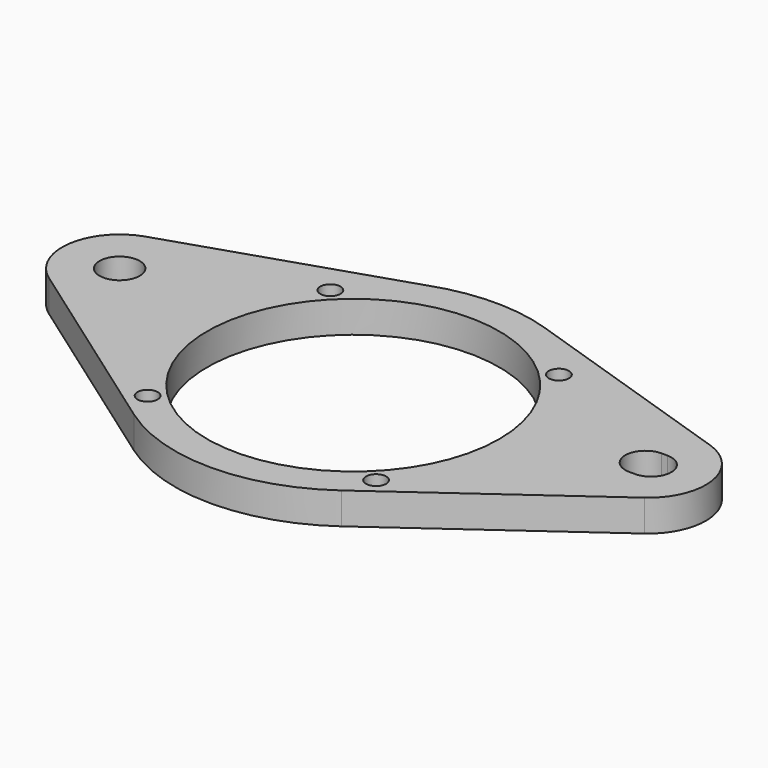
from build123d import *

# Parameters (mm, degrees)
F0_R      = 3.5
F0_R_2    = 25.4
F1_DEPTH  = 5.5
F2_DEPTH  = 33
F3_DEPTH  = 28
F4_R      = 2.5
F5_DEPTH  = 25.4
F6_R      = 5.08
F7_R      = 40.64
F8_DEPTH  = 33
F9_R      = 1.7526
F10_DEPTH = 5.501


with BuildPart() as f1:
    # F0 (on Top) → F1 (new body)
    with BuildSketch(Plane.XY):
        with BuildLine():
            Line((-3.3917498572, 9.4072330101), (-2.8084065037, 9.5975441082))
            ThreePointArc((-2.8084065037, 9.5975441082), (-3.1015382157, 9.5068638728), (-3.3917498572, 9.4072330101))
        make_face()
        with BuildLine():
            Line((35.7055754428, 22.1624223313), (-2.8084065037, 9.5975441082))
            Line((-2.8084065037, 9.5975441082), (-3.3917498572, 9.4072330101))
            ThreePointArc((-3.3917498572, 9.4072330101), (-9.9089012804, 1.3467276694), (-5.7794328291, -8.1607693371))
            Line((-5.7794328291, -8.1607693371), (28.3037582299, -32.2983849452))
            ThreePointArc((28.3037582299, -32.2983849452), (15.5024060308, -2.8251442248), (35.7055754428, 22.1624223313))
        make_face()
        Circle(F0_R, mode=Mode.SUBTRACT)
        with BuildLine():
            ThreePointArc((55.9525424009, 22.43259449), (45.80637798, 23.9972404711), (35.7055754428, 22.1624223313))
            ThreePointArc((35.7055754428, 22.1624223313), (15.5024060308, -2.8251442248), (28.3037582299, -32.2983849452))
            ThreePointArc((28.3037582299, -32.2983849452), (46.3284941146, -37.999810145), (64.3128808741, -32.1723590805))
            ThreePointArc((64.3128808741, -32.1723590805), (73.805134648, -21.1442690321), (77.22, -7))
            ThreePointArc((77.22, -7), (71.3467667481, 11.1561447666), (55.9525424009, 22.43259449))
        make_face()
        with Locations((46.22, -7)):
            Circle(F0_R_2, mode=Mode.SUBTRACT)
        with BuildLine():
            Line((95.0795298067, 9.4943853194), (55.9525424009, 22.43259449))
            ThreePointArc((55.9525424009, 22.43259449), (71.3467667481, 11.1561447666), (77.22, -7))
            ThreePointArc((77.22, -7), (73.805134648, -21.1442690321), (64.3128808741, -32.1723590805))
            Line((64.3128808741, -32.1723590805), (97.7764131852, -8.1201158324))
            ThreePointArc((97.7764131852, -8.1201158324), (101.8248141538, 1.5134229894), (95.0795298067, 9.4943853194))
        make_face()
        with BuildLine():
            ThreePointArc((91.44, -3.5), (87.94, 0), (91.44, 3.5))
            Line((91.44, 3.5), (92.44, 3.5))
            ThreePointArc((92.44, 3.5), (95.94, 0), (92.44, -3.5))
            Line((92.44, -3.5), (91.44, -3.5))
        make_face(mode=Mode.SUBTRACT)
    extrude(amount=F1_DEPTH)

    # F0 (on Top) → F2 (join)
    with BuildSketch(Plane.XY):
        with BuildLine():
            ThreePointArc((55.9525424009, 22.43259449), (45.80637798, 23.9972404711), (35.7055754428, 22.1624223313))
            ThreePointArc((35.7055754428, 22.1624223313), (15.5024060308, -2.8251442248), (28.3037582299, -32.2983849452))
            ThreePointArc((28.3037582299, -32.2983849452), (46.3284941146, -37.999810145), (64.3128808741, -32.1723590805))
            ThreePointArc((64.3128808741, -32.1723590805), (73.805134648, -21.1442690321), (77.22, -7))
            ThreePointArc((77.22, -7), (71.3467667481, 11.1561447666), (55.9525424009, 22.43259449))
        make_face()
        with Locations((46.22, -7)):
            Circle(F0_R_2, mode=Mode.SUBTRACT)
        with Locations((46.22, -7)):
            Circle(F0_R_2)
    extrude(amount=-F2_DEPTH)

    # F0 (on Top) → F3 (cut)
    with BuildSketch(Plane.XY):
        with Locations((46.22, -7)):
            Circle(F0_R_2)
    extrude(amount=-F3_DEPTH, mode=Mode.SUBTRACT)

    # F4 (on face) → F5 (cut)
    with BuildSketch(Plane(origin=(0, 0, -33), x_dir=(1, 0, 0), z_dir=(0, 0, -1))):
        with Locations((46.22, 7)):
            Circle(F4_R)
    extrude(amount=-F5_DEPTH, mode=Mode.SUBTRACT)

    # F6
    f6_edges = [f1.edges().sort_by_distance(p)[0] for p in [
        (36.487458, -36.432594, -33),
    ]]
    fillet(f6_edges, radius=F6_R)

    # F7 (on face) → F8 (cut, through all)
    with BuildSketch(Plane(origin=(0, 0, -33), x_dir=(1, 0, 0), z_dir=(0, 0, -1))):
        with Locations((46.22, 7)):
            Circle(F7_R)
    extrude(amount=-F8_DEPTH, mode=Mode.SUBTRACT)

    # F9 (on face) → F10 (cut, through all)
    with BuildSketch(Plane.XY.offset(5.5)):
        with Locations((26.3511833321, 12.8688166679)):
            Circle(F9_R)
        with Locations((26.3511833321, -26.8688166679)):
            Circle(F9_R)
        with Locations((66.0888166679, -26.8688166679)):
            Circle(F9_R)
        with Locations((66.0888166679, 12.8688166679)):
            Circle(F9_R)
    extrude(amount=-F10_DEPTH, mode=Mode.SUBTRACT)


solid = f1.part
